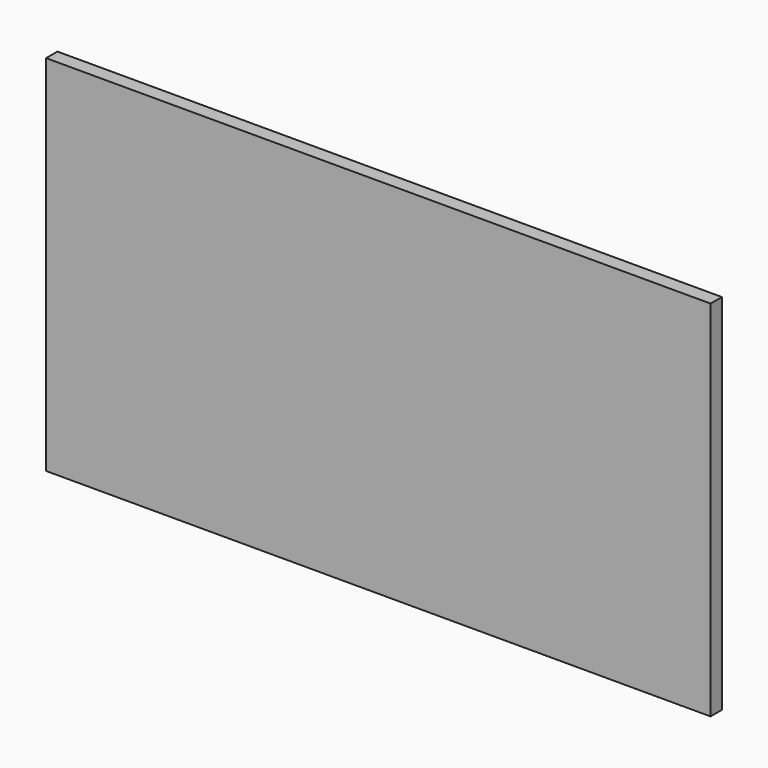
from build123d import *

# Parameters (mm, degrees)
F0_W     = 742.95
F0_H     = 406.4
F1_DEPTH = 15.875


# Not quite as in the source:
# - a length typed as a fraction of an inch, garbled in the dataset ("3 / 203.2 mm" for 3/8 in), is restored


with BuildPart() as f1:
    # F0 (on Front) → F1 (new body)
    with BuildSketch(Plane.XZ):
        with Locations((371.475, 203.2)):
            Rectangle(F0_W, F0_H)
    extrude(amount=F1_DEPTH)


solid = f1.part
